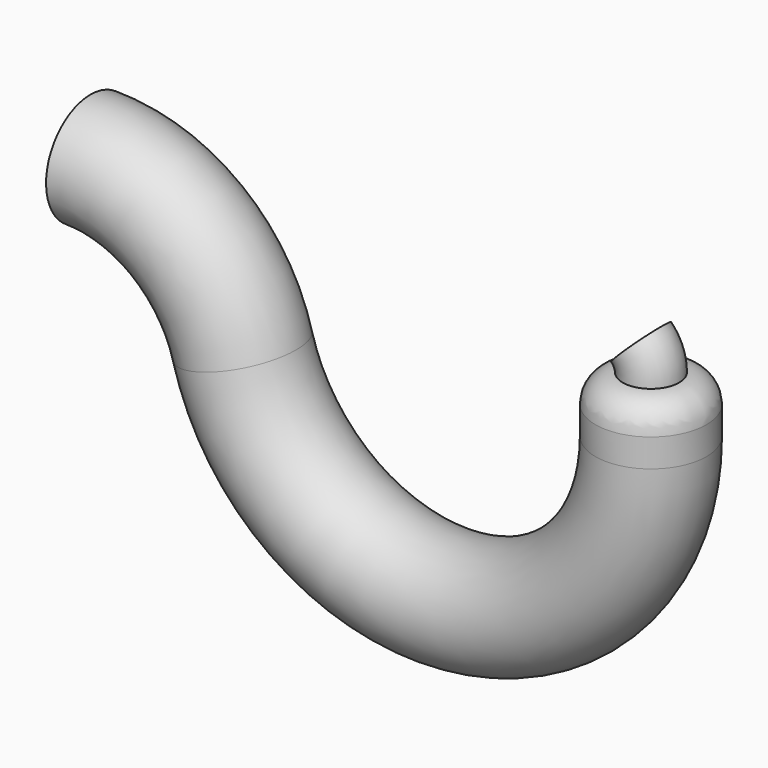
from build123d import *

# Parameters (mm, degrees)
F0_R     = 5
F1_ANGLE = 45
F3_R     = 9.8674102812
F3_R_2   = 5
F2_R     = 5
F4_DEPTH = 10
F6_R     = 9.8674102812
F7_ANGLE = 165
F8_R     = 9.8674102812
F9_ANGLE = 75


# Not quite as in the source:
# - a fillet or chamfer that OpenCascade refuses, or shapes differently, is made with other operations: its cross-section is extruded or revolved along the edge and cut away or added


with BuildPart() as f1:
    # F0 (on Top) → F1 (revolve)
    with BuildSketch(Plane.XY):
        with Locations((17.2625295818, 39.9485491216)):
            Circle(F0_R)
    revolve(axis=Axis((11.3439466804, 38.7977138162, 0), (0, -1, 0)), revolution_arc=F1_ANGLE)

    # F3 (on face) + F2 (on face) → F4 (join)
    with BuildSketch(Plane(origin=(0, 0, 0), x_dir=(1, 0, 0), z_dir=(0, 0, -1))):
        with Locations((17.2625295818, -39.9485491216)):
            Circle(F3_R)
        with Locations((17.2625295818, -39.9485491216)):
            Circle(F3_R_2, mode=Mode.SUBTRACT)
    with BuildSketch(Plane(origin=(0, 0, 0), x_dir=(1, 0, 0), z_dir=(0, 0, -1))):
        with Locations((17.2625295818, -39.9485491216)):
            Circle(F2_R)
    extrude(amount=F4_DEPTH)

    # F5: fillet of radius 5 on 1 edges, made by hand

    # F5_s1 → F5_t2 (revolve, cut)
    with BuildSketch(Plane.XZ.offset(-39.9485491216)):
        with BuildLine():
            ThreePointArc((27.129939863, -4.9982416875), (25.7120445931, -1.5099002903), (22.2625295818, 0))
            Line((22.2625295818, 0), (27.129939863, 0))
            Line((27.129939863, 0), (27.129939863, -4.9982416875))
        make_face()
    revolve(axis=Axis((17.2625295818, 39.9485491216, 0), (0, 0, -1)), mode=Mode.SUBTRACT)

    # F6 (on face) → F7 (revolve)
    with BuildSketch(Plane(origin=(0, 0, -10), x_dir=(1, 0, 0), z_dir=(0, 0, -1))):
        with Locations((17.2625295818, -39.9485491216)):
            Circle(F6_R)
    revolve(axis=Axis((-19.6528339293, 41.1798441783, -10), (0, 1, 0)), revolution_arc=F7_ANGLE)

    # F8 (on face) → F9 (revolve)
    with BuildSketch(Plane(origin=(1.1835097549, 0, -4.4169185366), x_dir=(0.9659258263, 0, 0.2588190451), z_dir=(-0.2588190451, 0, 0.9659258263))):
        with Locations((-58.4867338142, 39.9485491216)):
            Circle(F8_R)
    revolve(axis=Axis((-82.3409964635, 40.3092578053, -26.797242526), (0, -1, 0)), revolution_arc=F9_ANGLE)


solid = f1.part
